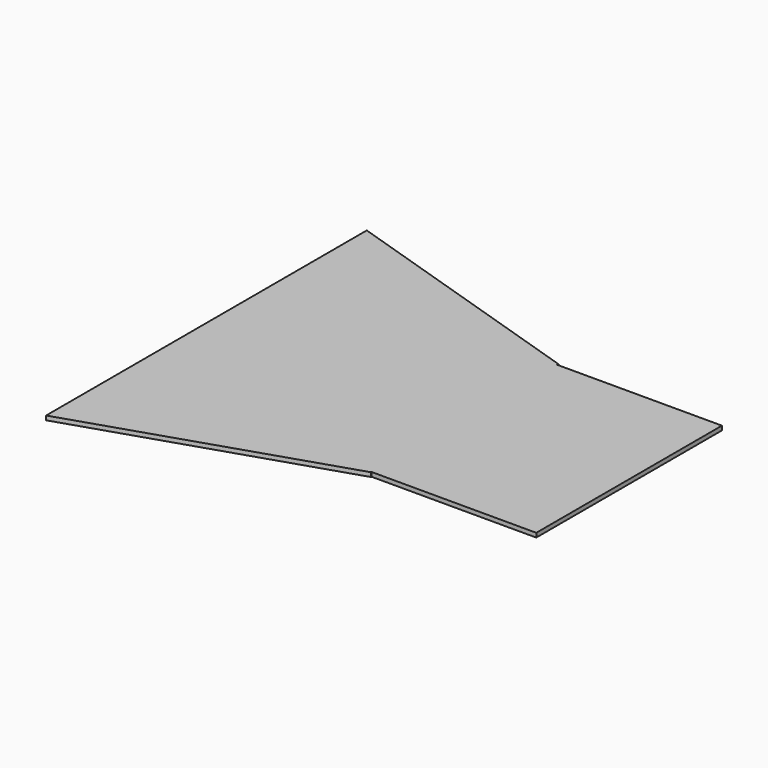
from build123d import *

# Parameters (mm, degrees)
F0_W     = 77.923713997
F0_H     = 109.7831092775
F1_DEPTH = 2


with BuildPart() as f1:
    # F0 (on Top) → F1 (new body)
    with BuildSketch(Plane.XY):
        Polygon((-98.5241234303, 94.8422709107), (-98.5241234303, 54.8422709107), (23.5521625727, 54.8422709107), (23.5521625727, 55.5602938927), align=None)
        Polygon((23.5521625727, 54.8422709107), (-98.5241234303, 54.8422709107), (-98.5241234303, -54.8019595444), (-98.5241234303, -54.9408383667), (23.5521625727, -54.9408383667), align=None)
        with Locations((62.5140195712, -0.049283728)):
            Rectangle(F0_W, F0_H)
        Polygon((23.5521625727, -55.2528910339), (23.5521625727, -54.9408383667), (-98.5241234303, -54.9408383667), (-98.5241234303, -94.7827324271), align=None)
    extrude(amount=F1_DEPTH)


solid = f1.part
